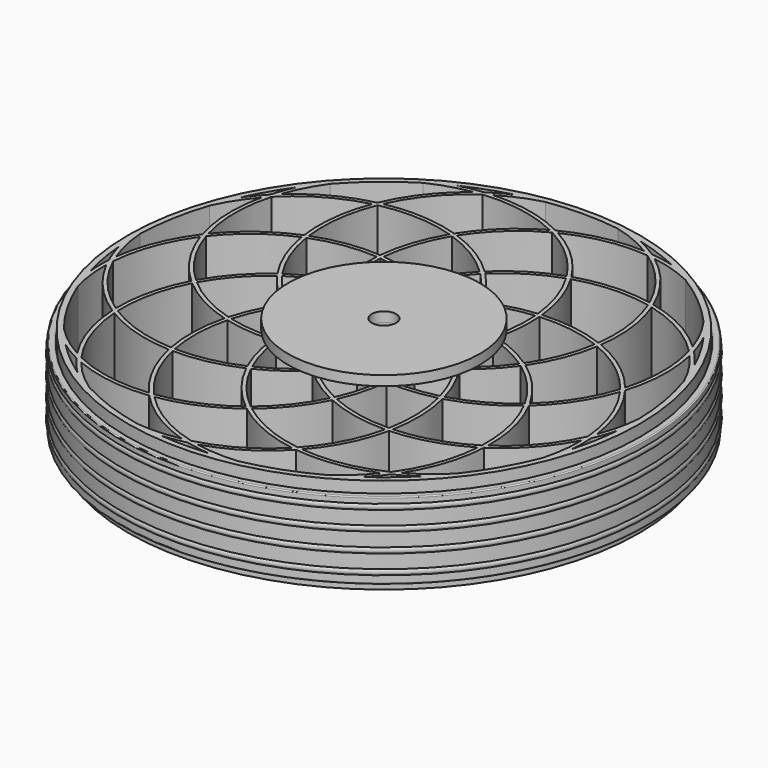
from build123d import *

# Parameters (mm, degrees)
F0_R      = 66.675
F0_R_2    = 65.175
F2_DEPTH  = 12.5
F1_R      = 39.0615311231
F1_R_2    = 38.0615311231
F3_DEPTH  = 12.5
F5_COUNT  = 9
F6_R      = 11.2255664066
F6_R_2    = 1.8415
F6_R_3    = 4.5
F7_DEPTH  = 12.5
F11_R     = 25
F11_R_2   = 4.5
F11_R_3   = 3.175
F12_DEPTH = 2.54
F13_DEPTH = 11.43


with BuildPart() as f2:
    # F0 (on Top) → F2 (new body, symmetric)
    with BuildSketch(Plane.XY):
        Circle(F0_R)
        Circle(F0_R_2, mode=Mode.SUBTRACT)
    extrude(amount=F2_DEPTH, both=True)

    # F1 (on Top) → F3 (join, symmetric)
    with BuildSketch(Plane.XY):
        with Locations((0, 27.6134688769)):
            Circle(F1_R)
        with Locations((0, 27.6134688769)):
            Circle(F1_R_2, mode=Mode.SUBTRACT)
    extrude(amount=F3_DEPTH, both=True)


with BuildPart() as f5_1:
    # F5: instance of F2
    add(f2.part.rotate(Axis((0, 0, -0.302568078), (0, 0, -1)), 1 * 360 / F5_COUNT))


with BuildPart() as f5_2:
    # F5: instance of F2
    add(f2.part.rotate(Axis((0, 0, -0.302568078), (0, 0, -1)), 2 * 360 / F5_COUNT))


with BuildPart() as f5_3:
    # F5: instance of F2
    add(f2.part.rotate(Axis((0, 0, -0.302568078), (0, 0, -1)), 3 * 360 / F5_COUNT))


with BuildPart() as f5_4:
    # F5: instance of F2
    add(f2.part.rotate(Axis((0, 0, -0.302568078), (0, 0, -1)), 4 * 360 / F5_COUNT))


with BuildPart() as f5_5:
    # F5: instance of F2
    add(f2.part.rotate(Axis((0, 0, -0.302568078), (0, 0, -1)), 5 * 360 / F5_COUNT))


with BuildPart() as f5_6:
    # F5: instance of F2
    add(f2.part.rotate(Axis((0, 0, -0.302568078), (0, 0, -1)), 6 * 360 / F5_COUNT))


with BuildPart() as f5_7:
    # F5: instance of F2
    add(f2.part.rotate(Axis((0, 0, -0.302568078), (0, 0, -1)), 7 * 360 / F5_COUNT))


with BuildPart() as f5_8:
    # F5: instance of F2
    add(f2.part.rotate(Axis((0, 0, -0.302568078), (0, 0, -1)), 8 * 360 / F5_COUNT))


with BuildPart() as f2_1:
    add(f2.part)

    add(f5_1.part)  # F7 merges F5_1

    add(f5_2.part)  # F7 merges F5_2

    add(f5_3.part)  # F7 merges F5_3

    add(f5_4.part)  # F7 merges F5_4

    add(f5_5.part)  # F7 merges F5_5

    add(f5_6.part)  # F7 merges F5_6

    add(f5_7.part)  # F7 merges F5_7

    add(f5_8.part)  # F7 merges F5_8
    # F6 (on Top) → F7 (join, symmetric)
    with BuildSketch(Plane.XY):
        Circle(F6_R)
        with Locations((-0.1832785542, -8.0035279239)):
            Circle(F6_R_2, mode=Mode.SUBTRACT)
        with Locations((7.9101246848, -0.093403239)):
            Circle(F6_R_2, mode=Mode.SUBTRACT)
        with Locations((-8.093403239, 0.0898753152)):
            Circle(F6_R_2, mode=Mode.SUBTRACT)
        Circle(F6_R_3, mode=Mode.SUBTRACT)
        with Locations((0, 8)):
            Circle(F6_R_2, mode=Mode.SUBTRACT)
    extrude(amount=F7_DEPTH, both=True)

    # F8: union 


with BuildPart() as f10:
    # F9 (on Front) → F10 (revolve)
    with BuildSketch(Plane.XZ):
        with BuildLine():
            Line((-68.3262243271, -10.271208613), (-67.0762243271, -10.271208613))
            ThreePointArc((-67.0762243271, -10.271208613), (-66.8994476318, -10.1979853083), (-66.8262243271, -10.021208613))
            Line((-66.8262243271, -10.021208613), (-66.8262243271, -8.2283153942))
            ThreePointArc((-66.8262243271, -8.2283153942), (-67.7012243271, -8.646208613), (-68.5762243271, -8.2283153942))
            Line((-68.5762243271, -8.2283153942), (-68.5762243271, -10.021208613))
            ThreePointArc((-68.5762243271, -10.021208613), (-68.5030010224, -10.1979853083), (-68.3262243271, -10.271208613))
        make_face()
        with BuildLine():
            ThreePointArc((-68.5762243271, -8.2283153942), (-67.7012243271, -8.646208613), (-66.8262243271, -8.2283153942))
            Line((-66.8262243271, -8.2283153942), (-66.8262243271, -6.8141018318))
            ThreePointArc((-66.8262243271, -6.8141018318), (-67.7012243271, -6.396208613), (-68.5762243271, -6.8141018318))
            Line((-68.5762243271, -6.8141018318), (-68.5762243271, -8.2283153942))
        make_face()
        with BuildLine():
            Line((-66.8262243271, -6.8141018318), (-66.8262243271, -8.2283153942))
            ThreePointArc((-66.8262243271, -8.2283153942), (-66.6405641553, -7.896208613), (-66.5762243271, -7.521208613))
            ThreePointArc((-66.5762243271, -7.521208613), (-66.6405641553, -7.146208613), (-66.8262243271, -6.8141018318))
        make_face()
        with BuildLine():
            ThreePointArc((-68.5762243271, -6.8141018318), (-68.8262243271, -7.521208613), (-68.5762243271, -8.2283153942))
            Line((-68.5762243271, -8.2283153942), (-68.5762243271, -6.8141018318))
        make_face()
        with BuildLine():
            ThreePointArc((-68.5762243271, -6.8141018318), (-67.7012243271, -6.396208613), (-66.8262243271, -6.8141018318))
            Line((-66.8262243271, -6.8141018318), (-66.8262243271, -3.2283153942))
            ThreePointArc((-66.8262243271, -3.2283153942), (-67.7012243271, -3.646208613), (-68.5762243271, -3.2283153942))
            Line((-68.5762243271, -3.2283153942), (-68.5762243271, -6.8141018318))
        make_face()
        with BuildLine():
            ThreePointArc((-68.5762243271, -3.2283153942), (-67.7012243271, -3.646208613), (-66.8262243271, -3.2283153942))
            Line((-66.8262243271, -3.2283153942), (-66.8262243271, -1.8141018318))
            ThreePointArc((-66.8262243271, -1.8141018318), (-67.7012243271, -1.396208613), (-68.5762243271, -1.8141018318))
            Line((-68.5762243271, -1.8141018318), (-68.5762243271, -3.2283153942))
        make_face()
        with BuildLine():
            Line((-66.8262243271, -1.8141018318), (-66.8262243271, -3.2283153942))
            ThreePointArc((-66.8262243271, -3.2283153942), (-66.6405641553, -2.896208613), (-66.5762243271, -2.521208613))
            ThreePointArc((-66.5762243271, -2.521208613), (-66.6405641553, -2.146208613), (-66.8262243271, -1.8141018318))
        make_face()
        with BuildLine():
            ThreePointArc((-68.5762243271, -1.8141018318), (-68.8262243271, -2.521208613), (-68.5762243271, -3.2283153942))
            Line((-68.5762243271, -3.2283153942), (-68.5762243271, -1.8141018318))
        make_face()
        with BuildLine():
            ThreePointArc((-68.5762243271, -1.8141018318), (-67.7012243271, -1.396208613), (-66.8262243271, -1.8141018318))
            Line((-66.8262243271, -1.8141018318), (-66.8262243271, 1.7716846058))
            ThreePointArc((-66.8262243271, 1.7716846058), (-67.7012243271, 1.353791387), (-68.5762243271, 1.7716846058))
            Line((-68.5762243271, 1.7716846058), (-68.5762243271, -1.8141018318))
        make_face()
        with BuildLine():
            ThreePointArc((-68.5762243271, 1.7716846058), (-67.7012243271, 1.353791387), (-66.8262243271, 1.7716846058))
            Line((-66.8262243271, 1.7716846058), (-66.8262243271, 3.1858981682))
            ThreePointArc((-66.8262243271, 3.1858981682), (-67.7012243271, 3.603791387), (-68.5762243271, 3.1858981682))
            Line((-68.5762243271, 3.1858981682), (-68.5762243271, 1.7716846058))
        make_face()
        with BuildLine():
            Line((-66.8262243271, 3.1858981682), (-66.8262243271, 1.7716846058))
            ThreePointArc((-66.8262243271, 1.7716846058), (-66.6405641553, 2.103791387), (-66.5762243271, 2.478791387))
            ThreePointArc((-66.5762243271, 2.478791387), (-66.6405641553, 2.853791387), (-66.8262243271, 3.1858981682))
        make_face()
        with BuildLine():
            ThreePointArc((-68.5762243271, 3.1858981682), (-68.8262243271, 2.478791387), (-68.5762243271, 1.7716846058))
            Line((-68.5762243271, 1.7716846058), (-68.5762243271, 3.1858981682))
        make_face()
        with BuildLine():
            ThreePointArc((-68.5762243271, 3.1858981682), (-67.7012243271, 3.603791387), (-66.8262243271, 3.1858981682))
            Line((-66.8262243271, 3.1858981682), (-66.8262243271, 6.7716846058))
            ThreePointArc((-66.8262243271, 6.7716846058), (-67.7012243271, 6.353791387), (-68.5762243271, 6.7716846058))
            Line((-68.5762243271, 6.7716846058), (-68.5762243271, 3.1858981682))
        make_face()
        with BuildLine():
            ThreePointArc((-68.5762243271, 6.7716846058), (-67.7012243271, 6.353791387), (-66.8262243271, 6.7716846058))
            Line((-66.8262243271, 6.7716846058), (-66.8262243271, 8.1858981682))
            ThreePointArc((-66.8262243271, 8.1858981682), (-67.7012243271, 8.603791387), (-68.5762243271, 8.1858981682))
            Line((-68.5762243271, 8.1858981682), (-68.5762243271, 6.7716846058))
        make_face()
        with BuildLine():
            Line((-66.8262243271, 8.1858981682), (-66.8262243271, 6.7716846058))
            ThreePointArc((-66.8262243271, 6.7716846058), (-66.6405641553, 7.103791387), (-66.5762243271, 7.478791387))
            ThreePointArc((-66.5762243271, 7.478791387), (-66.6405641553, 7.853791387), (-66.8262243271, 8.1858981682))
        make_face()
        with BuildLine():
            ThreePointArc((-68.5762243271, 8.1858981682), (-68.8262243271, 7.478791387), (-68.5762243271, 6.7716846058))
            Line((-68.5762243271, 6.7716846058), (-68.5762243271, 8.1858981682))
        make_face()
        with BuildLine():
            ThreePointArc((-68.5762243271, 8.1858981682), (-67.7012243271, 8.603791387), (-66.8262243271, 8.1858981682))
            Line((-66.8262243271, 8.1858981682), (-66.8262243271, 9.478791387))
            ThreePointArc((-66.8262243271, 9.478791387), (-66.8994476318, 9.6555680823), (-67.0762243271, 9.728791387))
            Line((-67.0762243271, 9.728791387), (-68.3262243271, 9.728791387))
            ThreePointArc((-68.3262243271, 9.728791387), (-68.5030010224, 9.6555680823), (-68.5762243271, 9.478791387))
            Line((-68.5762243271, 9.478791387), (-68.5762243271, 8.1858981682))
        make_face()
    revolve(axis=Axis((0, 0, 0), (0, 0, 1)))


with BuildPart() as f12:
    # F11 (on face) → F12 (new body)
    with BuildSketch(Plane.XY.offset(12.5)):
        Circle(F11_R)
        with BuildLine():
            ThreePointArc((-6.3795893863, -15.1704444884), (-10.1674555377, -16.1455325678), (-14.0353925659, -16.7267295138))
            ThreePointArc((-14.0353925659, -16.7267295138), (-14.1346855236, -12.8166313498), (-13.8321672776, -8.9169891285))
            ThreePointArc((-13.8321672776, -8.9169891285), (-11.3267805182, -9.7697794674), (-8.7693980651, -10.4509616489))
            ThreePointArc((-8.7693980651, -10.4509616489), (-7.6544797689, -12.8512056717), (-6.3795893863, -15.1704444884))
        make_face(mode=Mode.SUBTRACT)
        with BuildLine():
            ThreePointArc((4.8643247519, -15.7219557124), (2.589425471, -18.9037099464), (0, -21.835194634))
            ThreePointArc((0, -21.835194634), (-2.589425471, -18.9037099464), (-4.8643247519, -15.7219557124))
            ThreePointArc((-4.8643247519, -15.7219557124), (-2.3969240834, -14.7647994462), (0, -13.642761517))
            ThreePointArc((0, -13.642761517), (2.3969240834, -14.7647994462), (4.8643247519, -15.7219557124))
        make_face(mode=Mode.SUBTRACT)
        with BuildLine():
            ThreePointArc((-16.3277850068, 2.06033577), (-14.9567104654, -0.2033710967), (-13.4354973145, -2.3690406758))
            ThreePointArc((-13.4354973145, -2.3690406758), (-14.1242674672, -4.9243899382), (-14.6384227493, -7.5205136876))
            ThreePointArc((-14.6384227493, -7.5205136876), (-18.1668711017, -5.8326810631), (-21.5034689641, -3.7916417572))
            ThreePointArc((-21.5034689641, -3.7916417572), (-19.0661691302, -0.7325085036), (-16.3277850068, 2.06033577))
        make_face(mode=Mode.SUBTRACT)
        with BuildLine():
            ThreePointArc((6.3795893863, -15.1704444884), (7.6544797689, -12.8512056717), (8.7693980651, -10.4509616489))
            ThreePointArc((8.7693980651, -10.4509616489), (11.3267805182, -9.7697794674), (13.8321672776, -8.9169891285))
            ThreePointArc((13.8321672776, -8.9169891285), (14.1346855236, -12.8166313498), (14.0353925659, -16.7267295138))
            ThreePointArc((14.0353925659, -16.7267295138), (10.1674555377, -16.1455325678), (6.3795893863, -15.1704444884))
        make_face(mode=Mode.SUBTRACT)
        with BuildLine():
            ThreePointArc((16.3277850068, 2.06033577), (19.0661691302, -0.7325085036), (21.5034689641, -3.7916417572))
            ThreePointArc((21.5034689641, -3.7916417572), (18.1668711017, -5.8326810631), (14.6384227493, -7.5205136876))
            ThreePointArc((14.6384227493, -7.5205136876), (14.1242674672, -4.9243899382), (13.4354973145, -2.3690406758))
            ThreePointArc((13.4354973145, -2.3690406758), (14.9567104654, -0.2033710967), (16.3277850068, 2.06033577))
        make_face(mode=Mode.SUBTRACT)
        with BuildLine():
            ThreePointArc((-16.04777542, 3.6483490488), (-17.6658057749, 7.2093467341), (-18.9098332497, 10.917597317))
            ThreePointArc((-18.9098332497, 10.917597317), (-15.0763803039, 11.6943632123), (-11.1834506682, 12.0736066636))
            ThreePointArc((-11.1834506682, 12.0736066636), (-11.5882293605, 9.4581968703), (-11.8149780515, 6.8213807585))
            ThreePointArc((-11.8149780515, 6.8213807585), (-13.9851534439, 5.3066025759), (-16.04777542, 3.6483490488))
        make_face(mode=Mode.SUBTRACT)
        with BuildLine():
            ThreePointArc((-7.4680763983, 20.518371271), (-4.0321855781, 18.6493124129), (-0.8062554717, 16.4375028161))
            ThreePointArc((-0.8062554717, 16.4375028161), (-2.797486949, 14.6941694056), (-4.6660992494, 12.8200023247))
            ThreePointArc((-4.6660992494, 12.8200023247), (-7.3022306966, 13.0545767685), (-9.9481956205, 13.1101087184))
            ThreePointArc((-9.9481956205, 13.1101087184), (-8.8987135925, 16.8780410714), (-7.4680763983, 20.518371271))
        make_face(mode=Mode.SUBTRACT)
        Circle(F11_R_2, mode=Mode.SUBTRACT)
        with BuildLine():
            ThreePointArc((11.1834506682, 12.0736066636), (15.0763803039, 11.6943632123), (18.9098332497, 10.917597317))
            ThreePointArc((18.9098332497, 10.917597317), (17.6658057749, 7.2093467341), (16.04777542, 3.6483490488))
            ThreePointArc((16.04777542, 3.6483490488), (13.9851534439, 5.3066025759), (11.8149780515, 6.8213807585))
            ThreePointArc((11.8149780515, 6.8213807585), (11.5882293605, 9.4581968703), (11.1834506682, 12.0736066636))
        make_face(mode=Mode.SUBTRACT)
        with BuildLine():
            ThreePointArc((9.9481956205, 13.1101087184), (7.3022306966, 13.0545767685), (4.6660992494, 12.8200023247))
            ThreePointArc((4.6660992494, 12.8200023247), (2.797486949, 14.6941694056), (0.8062554717, 16.4375028161))
            ThreePointArc((0.8062554717, 16.4375028161), (4.0321855781, 18.6493124129), (7.4680763983, 20.518371271))
            ThreePointArc((7.4680763983, 20.518371271), (8.8987135925, 16.8780410714), (9.9481956205, 13.1101087184))
        make_face(mode=Mode.SUBTRACT)
        Circle(F11_R_2)
        Circle(F11_R_3, mode=Mode.SUBTRACT)
        with BuildLine():
            ThreePointArc((-14.6384227493, -7.5205136876), (-14.1242674672, -4.9243899382), (-13.4354973145, -2.3690406758))
            ThreePointArc((-13.4354973145, -2.3690406758), (-14.9567104654, -0.2033710967), (-16.3277850068, 2.06033577))
            ThreePointArc((-16.3277850068, 2.06033577), (-19.0661691302, -0.7325085036), (-21.5034689641, -3.7916417572))
            ThreePointArc((-21.5034689641, -3.7916417572), (-18.1668711017, -5.8326810631), (-14.6384227493, -7.5205136876))
        make_face()
        with BuildLine():
            ThreePointArc((-11.1834506682, 12.0736066636), (-15.0763803039, 11.6943632123), (-18.9098332497, 10.917597317))
            ThreePointArc((-18.9098332497, 10.917597317), (-17.6658057749, 7.2093467341), (-16.04777542, 3.6483490488))
            ThreePointArc((-16.04777542, 3.6483490488), (-13.9851534439, 5.3066025759), (-11.8149780515, 6.8213807585))
            ThreePointArc((-11.8149780515, 6.8213807585), (-11.5882293605, 9.4581968703), (-11.1834506682, 12.0736066636))
        make_face()
        with BuildLine():
            ThreePointArc((-4.6660992494, 12.8200023247), (-2.797486949, 14.6941694056), (-0.8062554717, 16.4375028161))
            ThreePointArc((-0.8062554717, 16.4375028161), (-4.0321855781, 18.6493124129), (-7.4680763983, 20.518371271))
            ThreePointArc((-7.4680763983, 20.518371271), (-8.8987135925, 16.8780410714), (-9.9481956205, 13.1101087184))
            ThreePointArc((-9.9481956205, 13.1101087184), (-7.3022306966, 13.0545767685), (-4.6660992494, 12.8200023247))
        make_face()
        with BuildLine():
            ThreePointArc((0.8062554717, 16.4375028161), (2.797486949, 14.6941694056), (4.6660992494, 12.8200023247))
            ThreePointArc((4.6660992494, 12.8200023247), (7.3022306966, 13.0545767685), (9.9481956205, 13.1101087184))
            ThreePointArc((9.9481956205, 13.1101087184), (8.8987135925, 16.8780410714), (7.4680763983, 20.518371271))
            ThreePointArc((7.4680763983, 20.518371271), (4.0321855781, 18.6493124129), (0.8062554717, 16.4375028161))
        make_face()
        with BuildLine():
            ThreePointArc((16.04777542, 3.6483490488), (17.6658057749, 7.2093467341), (18.9098332497, 10.917597317))
            ThreePointArc((18.9098332497, 10.917597317), (15.0763803039, 11.6943632123), (11.1834506682, 12.0736066636))
            ThreePointArc((11.1834506682, 12.0736066636), (11.5882293605, 9.4581968703), (11.8149780515, 6.8213807585))
            ThreePointArc((11.8149780515, 6.8213807585), (13.9851534439, 5.3066025759), (16.04777542, 3.6483490488))
        make_face()
        with BuildLine():
            ThreePointArc((14.6384227493, -7.5205136876), (18.1668711017, -5.8326810631), (21.5034689641, -3.7916417572))
            ThreePointArc((21.5034689641, -3.7916417572), (19.0661691302, -0.7325085036), (16.3277850068, 2.06033577))
            ThreePointArc((16.3277850068, 2.06033577), (14.9567104654, -0.2033710967), (13.4354973145, -2.3690406758))
            ThreePointArc((13.4354973145, -2.3690406758), (14.1242674672, -4.9243899382), (14.6384227493, -7.5205136876))
        make_face()
        with BuildLine():
            ThreePointArc((13.8321672776, -8.9169891285), (11.3267805182, -9.7697794674), (8.7693980651, -10.4509616489))
            ThreePointArc((8.7693980651, -10.4509616489), (7.6544797689, -12.8512056717), (6.3795893863, -15.1704444884))
            ThreePointArc((6.3795893863, -15.1704444884), (10.1674555377, -16.1455325678), (14.0353925659, -16.7267295138))
            ThreePointArc((14.0353925659, -16.7267295138), (14.1346855236, -12.8166313498), (13.8321672776, -8.9169891285))
        make_face()
        with BuildLine():
            ThreePointArc((-4.8643247519, -15.7219557124), (-2.589425471, -18.9037099464), (0, -21.835194634))
            ThreePointArc((0, -21.835194634), (2.589425471, -18.9037099464), (4.8643247519, -15.7219557124))
            ThreePointArc((4.8643247519, -15.7219557124), (2.3969240834, -14.7647994462), (0, -13.642761517))
            ThreePointArc((0, -13.642761517), (-2.3969240834, -14.7647994462), (-4.8643247519, -15.7219557124))
        make_face()
        with BuildLine():
            ThreePointArc((-13.8321672776, -8.9169891285), (-14.1346855236, -12.8166313498), (-14.0353925659, -16.7267295138))
            ThreePointArc((-14.0353925659, -16.7267295138), (-10.1674555377, -16.1455325678), (-6.3795893863, -15.1704444884))
            ThreePointArc((-6.3795893863, -15.1704444884), (-7.6544797689, -12.8512056717), (-8.7693980651, -10.4509616489))
            ThreePointArc((-8.7693980651, -10.4509616489), (-11.3267805182, -9.7697794674), (-13.8321672776, -8.9169891285))
        make_face()
    extrude(amount=F12_DEPTH)

    # F11 (on face) → F13 (join)
    with BuildSketch(Plane.XY.offset(12.5)):
        with BuildLine():
            ThreePointArc((-13.8321672776, -8.9169891285), (-14.1346855236, -12.8166313498), (-14.0353925659, -16.7267295138))
            ThreePointArc((-14.0353925659, -16.7267295138), (-10.1674555377, -16.1455325678), (-6.3795893863, -15.1704444884))
            ThreePointArc((-6.3795893863, -15.1704444884), (-7.6544797689, -12.8512056717), (-8.7693980651, -10.4509616489))
            ThreePointArc((-8.7693980651, -10.4509616489), (-11.3267805182, -9.7697794674), (-13.8321672776, -8.9169891285))
        make_face()
        with BuildLine():
            ThreePointArc((-14.6384227493, -7.5205136876), (-14.1242674672, -4.9243899382), (-13.4354973145, -2.3690406758))
            ThreePointArc((-13.4354973145, -2.3690406758), (-14.9567104654, -0.2033710967), (-16.3277850068, 2.06033577))
            ThreePointArc((-16.3277850068, 2.06033577), (-19.0661691302, -0.7325085036), (-21.5034689641, -3.7916417572))
            ThreePointArc((-21.5034689641, -3.7916417572), (-18.1668711017, -5.8326810631), (-14.6384227493, -7.5205136876))
        make_face()
        with BuildLine():
            ThreePointArc((-11.1834506682, 12.0736066636), (-15.0763803039, 11.6943632123), (-18.9098332497, 10.917597317))
            ThreePointArc((-18.9098332497, 10.917597317), (-17.6658057749, 7.2093467341), (-16.04777542, 3.6483490488))
            ThreePointArc((-16.04777542, 3.6483490488), (-13.9851534439, 5.3066025759), (-11.8149780515, 6.8213807585))
            ThreePointArc((-11.8149780515, 6.8213807585), (-11.5882293605, 9.4581968703), (-11.1834506682, 12.0736066636))
        make_face()
        with BuildLine():
            ThreePointArc((-4.6660992494, 12.8200023247), (-2.797486949, 14.6941694056), (-0.8062554717, 16.4375028161))
            ThreePointArc((-0.8062554717, 16.4375028161), (-4.0321855781, 18.6493124129), (-7.4680763983, 20.518371271))
            ThreePointArc((-7.4680763983, 20.518371271), (-8.8987135925, 16.8780410714), (-9.9481956205, 13.1101087184))
            ThreePointArc((-9.9481956205, 13.1101087184), (-7.3022306966, 13.0545767685), (-4.6660992494, 12.8200023247))
        make_face()
        with BuildLine():
            ThreePointArc((0.8062554717, 16.4375028161), (2.797486949, 14.6941694056), (4.6660992494, 12.8200023247))
            ThreePointArc((4.6660992494, 12.8200023247), (7.3022306966, 13.0545767685), (9.9481956205, 13.1101087184))
            ThreePointArc((9.9481956205, 13.1101087184), (8.8987135925, 16.8780410714), (7.4680763983, 20.518371271))
            ThreePointArc((7.4680763983, 20.518371271), (4.0321855781, 18.6493124129), (0.8062554717, 16.4375028161))
        make_face()
        with BuildLine():
            ThreePointArc((16.04777542, 3.6483490488), (17.6658057749, 7.2093467341), (18.9098332497, 10.917597317))
            ThreePointArc((18.9098332497, 10.917597317), (15.0763803039, 11.6943632123), (11.1834506682, 12.0736066636))
            ThreePointArc((11.1834506682, 12.0736066636), (11.5882293605, 9.4581968703), (11.8149780515, 6.8213807585))
            ThreePointArc((11.8149780515, 6.8213807585), (13.9851534439, 5.3066025759), (16.04777542, 3.6483490488))
        make_face()
        with BuildLine():
            ThreePointArc((14.6384227493, -7.5205136876), (18.1668711017, -5.8326810631), (21.5034689641, -3.7916417572))
            ThreePointArc((21.5034689641, -3.7916417572), (19.0661691302, -0.7325085036), (16.3277850068, 2.06033577))
            ThreePointArc((16.3277850068, 2.06033577), (14.9567104654, -0.2033710967), (13.4354973145, -2.3690406758))
            ThreePointArc((13.4354973145, -2.3690406758), (14.1242674672, -4.9243899382), (14.6384227493, -7.5205136876))
        make_face()
        with BuildLine():
            ThreePointArc((13.8321672776, -8.9169891285), (11.3267805182, -9.7697794674), (8.7693980651, -10.4509616489))
            ThreePointArc((8.7693980651, -10.4509616489), (7.6544797689, -12.8512056717), (6.3795893863, -15.1704444884))
            ThreePointArc((6.3795893863, -15.1704444884), (10.1674555377, -16.1455325678), (14.0353925659, -16.7267295138))
            ThreePointArc((14.0353925659, -16.7267295138), (14.1346855236, -12.8166313498), (13.8321672776, -8.9169891285))
        make_face()
        with BuildLine():
            ThreePointArc((-4.8643247519, -15.7219557124), (-2.589425471, -18.9037099464), (0, -21.835194634))
            ThreePointArc((0, -21.835194634), (2.589425471, -18.9037099464), (4.8643247519, -15.7219557124))
            ThreePointArc((4.8643247519, -15.7219557124), (2.3969240834, -14.7647994462), (0, -13.642761517))
            ThreePointArc((0, -13.642761517), (-2.3969240834, -14.7647994462), (-4.8643247519, -15.7219557124))
        make_face()
        Circle(F11_R_2)
        Circle(F11_R_3, mode=Mode.SUBTRACT)
    extrude(amount=-F13_DEPTH)


solid = Compound([f2_1.part, f10.part, f12.part])
